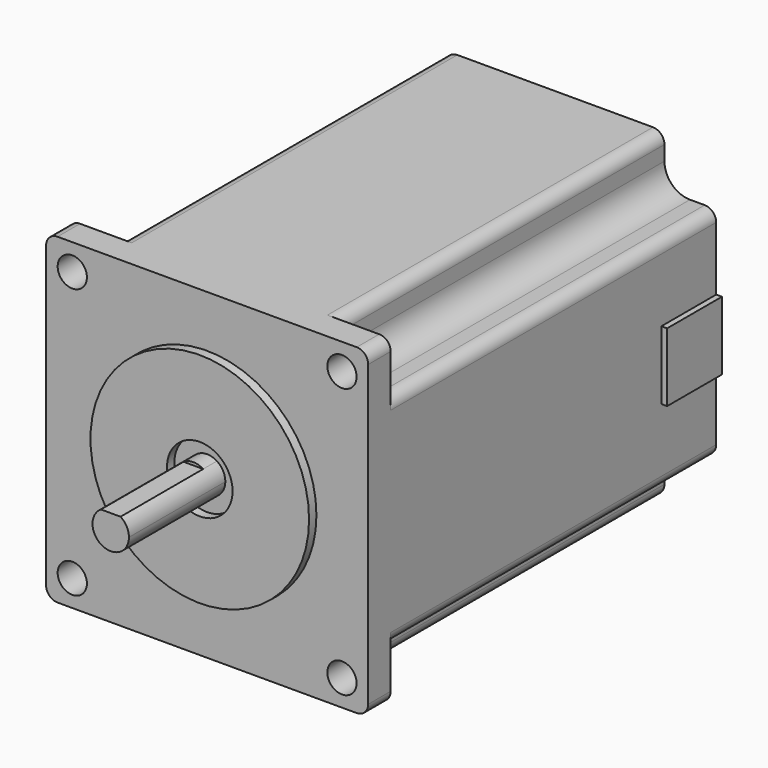
from build123d import *
from build123d import SkipClean  # not in build123d's __all__

# Parameters (mm, degrees)
F1_DEPTH      = 21
F2_DEPTH      = 3
F0_R          = 19.05
F0_R_2        = 5.715
F3_DEPTH      = 1.6
F3_DEPTH_BACK = 10
F0_W          = 56.134
F0_H          = 56.134
F0_R_3        = 2.55
F4_DEPTH      = 4.9022
F6_DEPTH      = 75.819
F7_R          = 2
F8_W          = 11.938
F8_H          = 11.938
F9_DEPTH      = 1


with BuildPart() as f1:
    # F0 (on Front) → F1 (new body)
    with BuildSketch(Plane.XZ):
        with BuildLine():
            ThreePointArc((-1.7102631376, 2.675), (-1.5248835264, -2.7848438432), (3.175, 0))
            ThreePointArc((3.175, 0), (2.7848438432, 1.5248835264), (1.7102631376, 2.675))
            Line((1.7102631376, 2.675), (-1.7102631376, 2.675))
        make_face()
    extrude(amount=F1_DEPTH)

    # F0 (on Front) → F2 (join, symmetric)
    with BuildSketch(Plane.XZ):
        with BuildLine():
            Line((-1.7102631376, 2.675), (1.7102631376, 2.675))
            ThreePointArc((1.7102631376, 2.675), (0, 3.175), (-1.7102631376, 2.675))
        make_face()
        with BuildLine():
            ThreePointArc((-1.7102631376, 2.675), (-1.5248835264, -2.7848438432), (3.175, 0))
            ThreePointArc((3.175, 0), (2.7848438432, 1.5248835264), (1.7102631376, 2.675))
            Line((1.7102631376, 2.675), (-1.7102631376, 2.675))
        make_face()
    with SkipClean():  # cleaning this boolean's faces spoils the solid; the shape is the same uncleaned
        extrude(amount=F2_DEPTH, both=True)



with BuildPart() as f3:
    # F0 (on Front) → F3 (new body, two sides)
    with BuildSketch(Plane.XZ) as f3_sk:
        Circle(F0_R)
        Circle(F0_R_2, mode=Mode.SUBTRACT)
    extrude(amount=F3_DEPTH)
    extrude(f3_sk.sketch, amount=-F3_DEPTH_BACK)

    # F0 (on Front) → F4 (join)
    with BuildSketch(Plane.XZ):
        Rectangle(F0_W, F0_H)
        with Locations((-23.5, -23.5)):
            Circle(F0_R_3, mode=Mode.SUBTRACT)
        with Locations((23.5, -23.5)):
            Circle(F0_R_3, mode=Mode.SUBTRACT)
        with Locations((-23.5, 23.5)):
            Circle(F0_R_3, mode=Mode.SUBTRACT)
        Circle(F0_R, mode=Mode.SUBTRACT)
        with Locations((23.5, 23.5)):
            Circle(F0_R_3, mode=Mode.SUBTRACT)
    extrude(amount=-F4_DEPTH)


with BuildPart() as f1_1:
    add(f1.part, clean=False)

    with SkipClean():  # cleaning this boolean's faces spoils the solid; the shape is the same uncleaned
        add(f3.part)  # F6 merges F3
    # F5 (on Front) → F6 (join)
    with BuildSketch(Plane.XZ):
        with BuildLine():
            ThreePointArc((-19.05, 23.5), (-20.3533748237, 20.3533748237), (-23.5, 19.05))
            Line((-23.5, 19.05), (-28.067, 19.05))
            Line((-28.067, 19.05), (-28.067, -19.05))
            Line((-28.067, -19.05), (-23.5, -19.05))
            ThreePointArc((-23.5, -19.05), (-20.3533748237, -20.3533748237), (-19.05, -23.5))
            Line((-19.05, -23.5), (-19.05, -28.067))
            Line((-19.05, -28.067), (19.05, -28.067))
            Line((19.05, -28.067), (19.05, -23.5))
            ThreePointArc((19.05, -23.5), (20.3533748237, -20.3533748237), (23.5, -19.05))
            Line((23.5, -19.05), (28.067, -19.05))
            Line((28.067, -19.05), (28.067, 19.05))
            Line((28.067, 19.05), (23.5, 19.05))
            ThreePointArc((23.5, 19.05), (20.3533748237, 20.3533748237), (19.05, 23.5))
            Line((19.05, 23.5), (19.05, 28.067))
            Line((19.05, 28.067), (-19.05, 28.067))
            Line((-19.05, 28.067), (-19.05, 23.5))
        make_face()
    with SkipClean():  # cleaning this boolean's faces spoils the solid; the shape is the same uncleaned
        extrude(amount=-F6_DEPTH)

    # F7
    f7_edges = [f1_1.edges().sort_by_distance(p)[0] for p in [
        (19.05, 40.3606, 28.067),
        (28.067, 40.3606, 19.05),
        (28.067, 2.4511, 28.067),
        (28.067, 2.4511, -28.067),
        (28.067, 40.3606, -19.05),
        (19.05, 40.3606, -28.067),
        (-19.05, 40.3606, -28.067),
        (-28.067, 40.3606, -19.05),
        (-28.067, 2.4511, -28.067),
        (-28.067, 2.4511, 28.067),
        (-28.067, 40.3606, 19.05),
        (-19.05, 40.3606, 28.067),
    ]]
    fillet(f7_edges, radius=F7_R)

    # F8 (on face) → F9 (join)
    with BuildSketch(Plane.YZ.offset(28.067)):
        with Locations((69.85, 0)):
            Rectangle(F8_W, F8_H)
    extrude(amount=F9_DEPTH)


solid = f1_1.part
